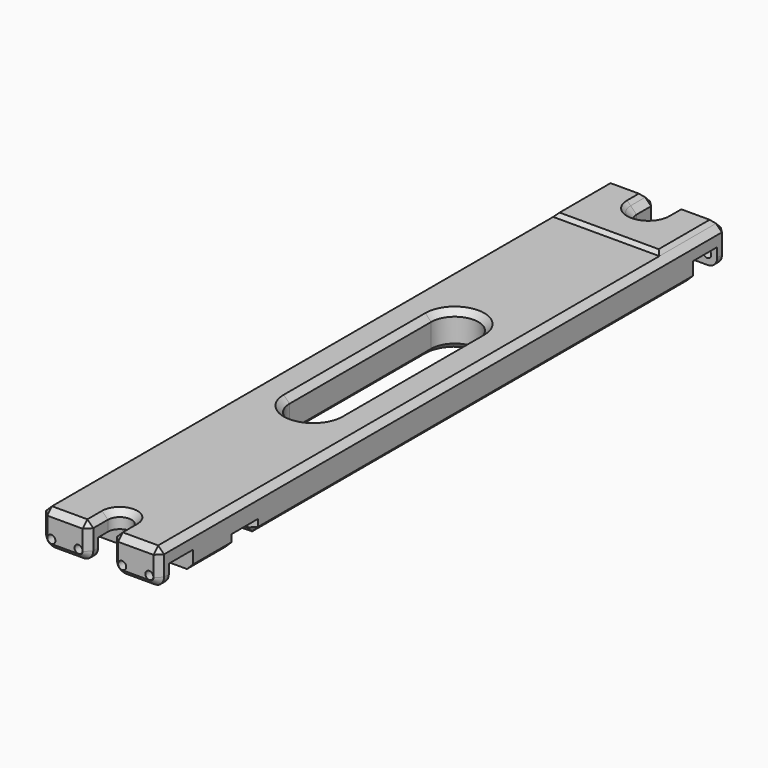
from build123d import *

# Parameters (mm, degrees)
F1_DEPTH       = 50
F3_DEPTH       = 30.001
F6_D           = 6.8
F6_DEPTH       = 13.75
F6_TIP         = 2.0429261047
F6_ON_F4_D     = 6.8
F6_ON_F4_DEPTH = 13.75
F6_ON_F4_TIP   = 2.0429261047
F7_D           = 3.3
F7_DEPTH       = 16.1
F7_START       = 35.5
F7_TIP         = 0.9914200214
F7_ON_F4_D     = 3.3
F7_ON_F4_DEPTH = 16.1
F7_ON_F4_START = 35.5
F7_ON_F4_TIP   = 0.9914200214
F9_D           = 3.3
F9_DEPTH       = 10.1
F9_TIP         = 0.9914200214
F11_DEPTH      = 11
F12_D          = 5
F12_DEPTH      = 15
F12_START      = 11
F12_TIP        = 1.5021515476
F13_R          = 8
F14_SIZE       = 5
F16_DEPTH      = 3
F17_SIZE       = 2.99999


# Not quite as in the source:
# - a fillet or chamfer is up to 0.001 mm smaller than in the source, because OpenCascade refuses the exact size


with BuildPart() as f1:
    # F0 (on Right) → F1 (new body, symmetric)
    with BuildSketch(Plane.YZ):
        Polygon((-300.5, 0), (-300.5, -30), (-290.5, -30), (-290.5, -14), (-265, -14), (-265, -30), (265, -30), (265, -14), (290.5, -14), (290.5, -30), (300.5, -30), (300.5, 0), align=None)
    extrude(amount=F1_DEPTH, both=True)

    # F2 (on face) → F3 (cut, through all)
    with BuildSketch(Plane.XY):
        with BuildLine():
            ThreePointArc((-20, -75), (0, -95), (20, -75))
            Line((20, -75), (-20, -75))
        make_face()
        with BuildLine():
            ThreePointArc((-20, -75), (0, -55), (20, -75))
            Line((20, -75), (20, 75))
            ThreePointArc((20, 75), (0, 55), (-20, 75))
            Line((-20, 75), (-20, -75))
        make_face()
        with BuildLine():
            Line((-20, -75), (20, -75))
            ThreePointArc((20, -75), (0, -55), (-20, -75))
        make_face()
        with BuildLine():
            ThreePointArc((-20, 75), (0, 55), (20, 75))
            Line((20, 75), (-20, 75))
        make_face()
        with BuildLine():
            Line((-20, 75), (20, 75))
            ThreePointArc((20, 75), (0, 95), (-20, 75))
        make_face()
        with BuildLine():
            Line((-10, 280), (10, 280))
            ThreePointArc((10, 280), (0, 290), (-10, 280))
        make_face()
        with BuildLine():
            ThreePointArc((-10, 280), (0, 270), (10, 280))
            Line((10, 280), (-10, 280))
        make_face()
        with BuildLine():
            ThreePointArc((-10, 280), (0, 290), (10, 280))
            Line((10, 280), (10, 300.5))
            Line((10, 300.5), (-10, 300.5))
            Line((-10, 300.5), (-10, 280))
        make_face()
        with BuildLine():
            Line((-10, -280), (10, -280))
            ThreePointArc((10, -280), (0, -270), (-10, -280))
        make_face()
        with BuildLine():
            Line((10, -300.5), (10, -280))
            ThreePointArc((10, -280), (0, -290), (-10, -280))
            Line((-10, -280), (-10, -300.5))
            Line((-10, -300.5), (10, -300.5))
        make_face()
        with BuildLine():
            ThreePointArc((-10, -280), (0, -290), (10, -280))
            Line((10, -280), (-10, -280))
        make_face()
    extrude(amount=-F3_DEPTH, mode=Mode.SUBTRACT)

    # F6
    with Locations(Plane.XZ.offset(300.5)):
        with Locations((-41.5, -21.5), (-18.5, -21.5), (18.5, -21.5), (41.5, -21.5)):
            Hole(F6_D / 2, depth=F6_DEPTH)
            with Locations((0, 0, -(F6_DEPTH + F6_TIP / 2))):  # 118° drill point
                Cone(0, F6_D / 2, F6_TIP, mode=Mode.SUBTRACT)

    # F6 on F4
    with Locations(Plane(origin=(0, 300.5, 0), x_dir=(-1, 0, 0), z_dir=(0, 1, 0))):
        with Locations((-41.5, -21.5), (-18.5, -21.5), (18.5, -21.5), (41.5, -21.5)):
            Hole(F6_ON_F4_D / 2, depth=F6_ON_F4_DEPTH)
            with Locations((0, 0, -(F6_ON_F4_DEPTH + F6_ON_F4_TIP / 2))):  # 118° drill point
                Cone(0, F6_ON_F4_D / 2, F6_ON_F4_TIP, mode=Mode.SUBTRACT)

    # F7
    # its depths count from where the whole tool has entered the part; down to there all is cleared
    with Locations(Plane.XZ.offset(300.5)):
        with Locations((0, -24.25)):
            Hole(F7_D / 2, depth=F7_START)
    with Locations(Plane.XZ.offset(300.5).offset(-F7_START)):
        with Locations((0, -24.25)):
            Hole(F7_D / 2, depth=F7_DEPTH)
            with Locations((0, 0, -(F7_DEPTH + F7_TIP / 2))):  # 118° drill point
                Cone(0, F7_D / 2, F7_TIP, mode=Mode.SUBTRACT)

    # F7 on F4
    # its depths count from where the whole tool has entered the part; down to there all is cleared
    with Locations(Plane(origin=(0, 300.5, 0), x_dir=(-1, 0, 0), z_dir=(0, 1, 0))):
        with Locations((0, -24.25)):
            Hole(F7_ON_F4_D / 2, depth=F7_ON_F4_START)
    with Locations(Plane(origin=(0, 300.5, 0), x_dir=(-1, 0, 0), z_dir=(0, 1, 0)).offset(-F7_ON_F4_START)):
        with Locations((0, -24.25)):
            Hole(F7_ON_F4_D / 2, depth=F7_ON_F4_DEPTH)
            with Locations((0, 0, -(F7_ON_F4_DEPTH + F7_ON_F4_TIP / 2))):  # 118° drill point
                Cone(0, F7_ON_F4_D / 2, F7_ON_F4_TIP, mode=Mode.SUBTRACT)

    # F9
    with Locations(Plane(origin=(0, 0, -14), x_dir=(1, 0, 0), z_dir=(0, 0, -1))):
        with Locations((-40, 280.25), (-20, 280.25), (20, 280.25), (40, 280.25), (-40, -280.25), (-20, -280.25), (20, -280.25), (40, -280.25)):
            Hole(F9_D / 2, depth=F9_DEPTH)
            with Locations((0, 0, -(F9_DEPTH + F9_TIP / 2))):  # 118° drill point
                Cone(0, F9_D / 2, F9_TIP, mode=Mode.SUBTRACT)

    # F10 (on face) → F11 (cut)
    with BuildSketch(Plane(origin=(0, 0, -30), x_dir=(1, 0, 0), z_dir=(0, 0, -1))):
        with BuildLine():
            Line((40, 201), (40, 219))
            ThreePointArc((40, 219), (31, 210), (40, 201))
        make_face()
        with BuildLine():
            ThreePointArc((40, 201), (46.3639610307, 203.6360389693), (49, 210))
            ThreePointArc((49, 210), (46.3639610307, 216.3639610307), (40, 219))
            Line((40, 219), (40, 201))
        make_face()
        with BuildLine():
            ThreePointArc((40, 219), (46.3639610307, 216.3639610307), (49, 210))
            ThreePointArc((49, 210), (46.3639610307, 203.6360389693), (40, 201))
            Line((40, 201), (50, 201))
            Line((50, 201), (50, 219))
            Line((50, 219), (40, 219))
        make_face()
    extrude(amount=-F11_DEPTH, mode=Mode.SUBTRACT)

    # F12
    # its depths count from where the whole tool has entered the part; down to there all is cleared
    with Locations(Plane(origin=(0, 0, -30), x_dir=(1, 0, 0), z_dir=(0, 0, -1)).offset(-F12_START)):
        with Locations((40, 210)):
            Hole(F12_D / 2, depth=F12_DEPTH)
            with Locations((0, 0, -(F12_DEPTH + F12_TIP / 2))):  # 118° drill point
                Cone(0, F12_D / 2, F12_TIP, mode=Mode.SUBTRACT)

    # F13
    f13_edges = [f1.edges().sort_by_distance(p)[0] for p in [
        (10, -295.5, -30),
        (50, -295.5, -30),
        (-50, -295.5, -30),
        (-10, -295.5, -30),
        (-50, 295.5, -30),
        (-10, 295.5, -30),
        (50, 295.5, -30),
        (10, 295.5, -30),
    ]]
    fillet(f13_edges, radius=F13_R)

    # F14
    f14_edges = [f1.edges().sort_by_distance(p)[0] for p in [
        (10, 300.5, -11),
        (-10, 300.5, -11),
        (10, -300.5, -11),
        (-10, -300.5, -11),
        (50, -219, -24.5),
        (50, -201, -24.5),
        (-50, 0, -30),
        (50, -242, -30),
        (50, 32, -30),
        (0, 95, -30),
        (31, -210, -30),
        (-30, -300.5, 0),
        (30, -300.5, 0),
        (10, -290.25, 0),
        (-30, 300.5, 0),
        (-10, 290.25, 0),
        (0, 270, 0),
        (10, 290.25, 0),
        (30, 300.5, 0),
        (50, 0, 0),
        (0, -270, 0),
        (-10, -290.25, 0),
        (-50, 0, 0),
        (0, -95, 0),
        (20, 0, 0),
        (0, 95, 0),
        (-20, 0, 0),
    ]]
    chamfer(f14_edges, length=F14_SIZE)


with BuildPart() as f16:
    # F15 (on face) → F16 (new body)
    with BuildSketch(Plane.XY):
        with BuildLine():
            Line((-15, 295.5), (-45, 295.5))
            Line((-45, 295.5), (-45, 235.5))
            Line((-45, 235.5), (45, 235.5))
            Line((45, 235.5), (45, 295.5))
            Line((45, 295.5), (15, 295.5))
            Line((15, 295.5), (15, 280))
            ThreePointArc((15, 280), (0, 265), (-15, 280))
            Line((-15, 280), (-15, 295.5))
        make_face()
    extrude(amount=F16_DEPTH)

    # F17 (size 3 in the source; OpenCascade refuses exactly that, so slightly less here)
    f17_edges = [f16.edges().sort_by_distance(p)[0] for p in [
        (0, 235.5, 3),
        (0, 265, 3),
        (45, 265.5, 3),
        (-15, 287.75, 3),
        (-30, 295.5, 3),
        (-45, 265.5, 3),
        (30, 295.5, 3),
        (15, 287.75, 3),
    ]]
    chamfer(f17_edges, length=F17_SIZE)


solid = Compound([f1.part, f16.part])
